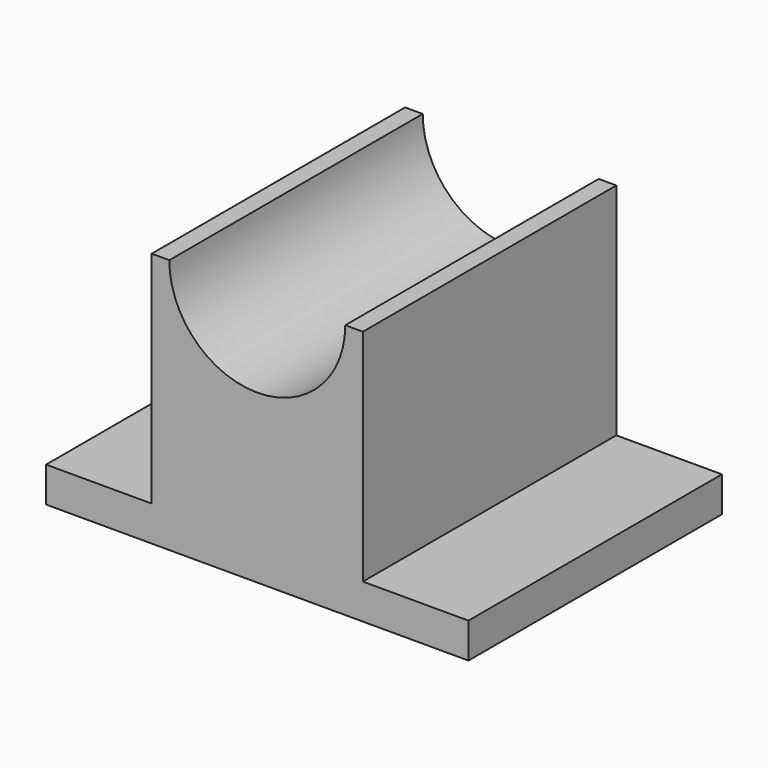
from build123d import *

# Parameters (mm, degrees)
F1_DEPTH = 114.3


# Not quite as in the source:
# - a feature names something its author has since deleted; it is built from what else it names


with BuildPart() as f1:
    # F0 (on Front) → F1 (new body)
    with BuildSketch(Plane.XZ):
        with BuildLine():
            Line((0, 12.7), (0, 0))
            Line((0, 0), (152.4, 0))
            Line((152.4, 0), (152.4, 12.7))
            Line((152.4, 12.7), (114.3, 12.7))
            Line((114.3, 12.7), (114.3, 92.075))
            Line((114.3, 92.075), (107.95, 92.075))
            ThreePointArc((107.95, 92.075), (76.2, 60.325), (44.45, 92.075))
            Line((44.45, 92.075), (38.1, 92.075))
            Line((38.1, 92.075), (38.1, 12.7))
            Line((38.1, 12.7), (0, 12.7))
        make_face()
    extrude(amount=F1_DEPTH)


solid = f1.part
